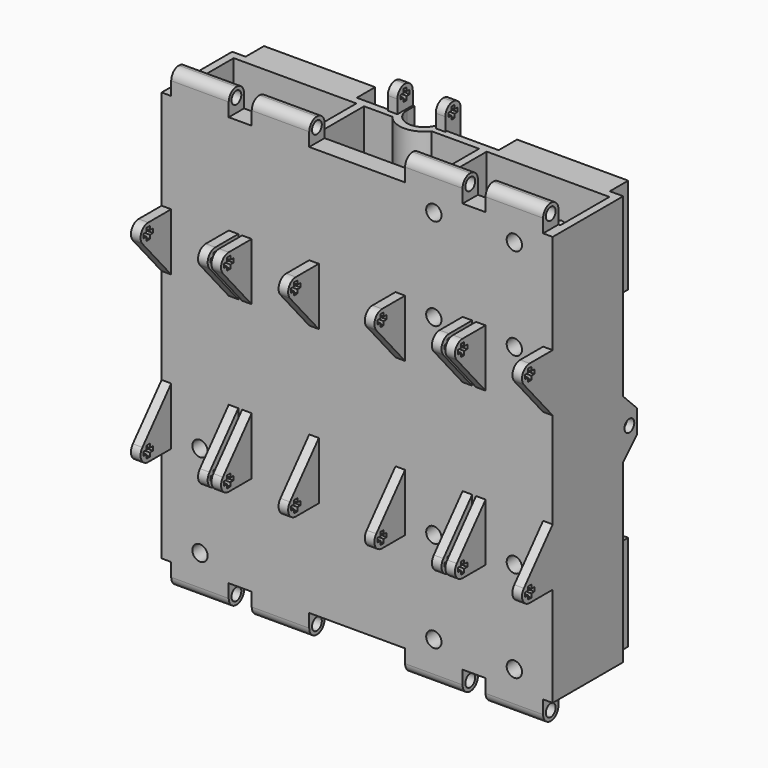
from build123d import *

# Parameters (mm, degrees)
F0_W      = 50.8
F0_H      = 25.4
F1_DEPTH  = 39.6875
F2_R      = 4.7625
F3_DEPTH  = 38.1
F5_DEPTH  = 39.6875
F6_W      = 3.96875
F6_H      = 7.9375
F7_DEPTH  = 9.525
F8_W      = 23.8125
F8_H      = 7.9375
F9_DEPTH  = 9.525
F11_DEPTH = 90.4875
F13_DEPTH = 39.6875
F14_W     = 23.8125
F14_H     = 7.9375
F14_W_2   = 3.96875
F15_DEPTH = 9.525
F16_W     = 3.96875
F16_H     = 23.8125
F17_DEPTH = 25.4
F18_R     = 3.96874
F19_R     = 3.175
F20_DEPTH = 7.9375
F21_R     = 2.54
F21_W     = 1.56845
F21_H     = 1.6891
F21_W_2   = 1.6891
F21_H_2   = 1.56845
F22_DEPTH = 161.925
F23_R     = 4.7625
F24_DEPTH = 38.1
F25_R     = 0.79375
F26_DEPTH = 3.175
F27_R     = 0.79375
F28_DEPTH = 6.35
F30_DEPTH = 39.6875
F31_R     = 1.5875
F31_R_2   = 0.79375
F32_DEPTH = 4.7625
F33_DEPTH = 3.175
F34_DEPTH = 3.175
F36_DEPTH = 161.925


# Not quite as in the source:
# - a fillet or chamfer is up to 0.001 mm smaller than in the source, because OpenCascade refuses the exact size
# - a feature names something its author has since deleted; it is built from what else it names


with BuildPart() as f1:
    # F0 (on Top) → F1 (new body)
    with BuildSketch(Plane.XY):
        Polygon((-3.175, 28.575), (-3.175, -7.9375), (158.75, -7.9375), (158.75, 28.575), (153.19375, 28.575), (153.19375, 38.1), (107.15625, 38.1), (107.15625, 28.575), (93.6625, 28.575), (93.6625, 35.71875), (69.85, 35.71875), (69.85, 28.575), (48.41875, 28.575), (48.41875, 38.1), (2.38125, 38.1), (2.38125, 28.575), align=None)
        with Locations((25.4, 12.7)):
            Rectangle(F0_W, F0_H, mode=Mode.SUBTRACT)
        Polygon((53.975, 0), (53.975, 25.4), (69.85, 25.4), (69.85, 11.6781862453), (93.6625, 11.6781862453), (93.6625, 25.4), (101.6, 25.4), (101.6, 0), align=None, mode=Mode.SUBTRACT)
        with Locations((130.175, 12.7)):
            Rectangle(F0_W, F0_H, mode=Mode.SUBTRACT)
    extrude(amount=F1_DEPTH)

    # F2 (on face) → F3 (cut)
    with BuildSketch(Plane.XY.offset(39.6875)):
        with Locations((146.84375, 31.75)):
            Circle(F2_R)
        with Locations((135.73125, 31.75)):
            Circle(F2_R)
        with Locations((113.50625, 31.75)):
            Circle(F2_R)
        with Locations((124.61875, 31.75)):
            Circle(F2_R)
        with Locations((8.73125, 31.75)):
            Circle(F2_R)
        with Locations((19.84375, 31.75)):
            Circle(F2_R)
        with Locations((30.95625, 31.75)):
            Circle(F2_R)
        with Locations((42.06875, 31.75)):
            Circle(F2_R)
    extrude(amount=-F3_DEPTH, mode=Mode.SUBTRACT)

    # F4 (on face) → F5 (cut, through all)
    with BuildSketch(Plane(origin=(0, 0, 0), x_dir=(1, 0, 0), z_dir=(0, 0, -1))):
        with BuildLine():
            Line((74.6125, -35.71875), (88.9, -35.71875))
            Line((88.9, -35.71875), (88.9, -31.75))
            ThreePointArc((88.9, -31.75), (81.75625, -24.60625), (74.6125, -31.75))
            Line((74.6125, -31.75), (74.6125, -35.71875))
        make_face()
        with BuildLine():
            Line((89.8897671705, -25.4), (93.6625, -25.4))
            Line((93.6625, -25.4), (93.6625, -11.6781862453))
            Line((93.6625, -11.6781862453), (69.85, -11.6781862453))
            Line((69.85, -11.6781862453), (69.85, -25.4))
            Line((69.85, -25.4), (73.6227328295, -25.4))
            ThreePointArc((73.6227328295, -25.4), (81.75625, -21.43125), (89.8897671705, -25.4))
        make_face()
    extrude(amount=-F5_DEPTH, mode=Mode.SUBTRACT)

    # F6 (on face) → F7 (join)
    with BuildSketch(Plane(origin=(0, 0, 0), x_dir=(1, 0, 0), z_dir=(0, 0, -1))):
        with Locations((91.678125, -31.75)):
            Rectangle(F6_W, F6_H)
        with Locations((71.834375, -31.75)):
            Rectangle(F6_W, F6_H)
    extrude(amount=F7_DEPTH)

    # F8 (on face) → F9 (join)
    with BuildSketch(Plane(origin=(0, 0, 0), x_dir=(1, 0, 0), z_dir=(0, 0, -1))):
        with Locations((142.875, 3.96875)):
            Rectangle(F8_W, F8_H)
        with Locations((12.7, 3.96875)):
            Rectangle(F8_W, F8_H)
        with Locations((109.5375, 3.96875)):
            Rectangle(F8_W, F8_H)
        with Locations((46.0375, 3.96875)):
            Rectangle(F8_W, F8_H)
    extrude(amount=F9_DEPTH)

    # F10 (on face) → F11 (join)
    with BuildSketch(Plane.XY.offset(39.6875)):
        Polygon((0, 0), (0, 35.71875), (-3.175, 35.71875), (-3.175, -7.9375), (158.75, -7.9375), (158.75, 35.71875), (155.575, 35.71875), (155.575, 0), (104.775, 0), (104.775, 35.71875), (101.6, 35.71875), (101.6, 0), (53.975, 0), (53.975, 35.71875), (50.8, 35.71875), (50.8, 0), align=None)
    extrude(amount=F11_DEPTH)

    # F12 (on face) → F13 (join)
    with BuildSketch(Plane.XY.offset(130.175)):
        Polygon((155.575, 25.4), (155.575, 28.575), (153.19375, 28.575), (153.19375, 38.1), (107.15625, 38.1), (107.15625, 28.575), (104.775, 28.575), (104.775, 25.4), align=None)
        Polygon((61.9125, 28.575), (53.975, 28.575), (53.975, 25.4), (61.9125, 25.4), (61.9125, 11.6781862453), (85.725, 11.6781862453), (85.725, 25.4), (101.6, 25.4), (101.6, 28.575), (85.725, 28.575), (85.725, 35.71875), (61.9125, 35.71875), align=None)
        Polygon((-3.175, 28.575), (-3.175, -7.9375), (158.75, -7.9375), (158.75, 28.575), (155.575, 28.575), (155.575, 25.4), (155.575, 0), (104.775, 0), (104.775, 25.4), (104.775, 28.575), (101.6, 28.575), (101.6, 25.4), (101.6, 0), (53.975, 0), (53.975, 25.4), (53.975, 28.575), (50.8, 28.575), (50.8, 25.4), (50.8, 0), (0, 0), (0, 25.4), (0, 28.575), align=None)
        Polygon((2.38125, 28.575), (0, 28.575), (0, 25.4), (50.8, 25.4), (50.8, 28.575), (48.41875, 28.575), (48.41875, 38.1), (2.38125, 38.1), align=None)
    extrude(amount=F13_DEPTH)

    # F14 (on face) → F15 (join)
    with BuildSketch(Plane.XY.offset(169.8625)):
        with Locations((12.7, -3.96875)):
            Rectangle(F14_W, F14_H)
        with Locations((109.5375, -3.96875)):
            Rectangle(F14_W, F14_H)
        with Locations((142.875, -3.96875)):
            Rectangle(F14_W, F14_H)
        with Locations((46.0375, -3.96875)):
            Rectangle(F14_W, F14_H)
        with Locations((63.896875, 31.75)):
            Rectangle(F14_W_2, F14_H)
        with Locations((83.740625, 31.75)):
            Rectangle(F14_W_2, F14_H)
    extrude(amount=F15_DEPTH)

    # F16 (on face) → F17 (join)
    with BuildSketch(Plane.XZ.offset(7.9375)):
        with Locations((156.765625, 53.18125)):
            Rectangle(F16_W, F16_H)
        with Locations((128.984375, 53.18125)):
            Rectangle(F16_W, F16_H)
        with Locations((26.590625, 53.18125)):
            Rectangle(F16_W, F16_H)
        with Locations((-1.190625, 53.18125)):
            Rectangle(F16_W, F16_H)
        with Locations((59.928125, 53.18125)):
            Rectangle(F16_W, F16_H)
        with Locations((32.146875, 53.18125)):
            Rectangle(F16_W, F16_H)
        with Locations((123.428125, 53.18125)):
            Rectangle(F16_W, F16_H)
        with Locations((95.646875, 53.18125)):
            Rectangle(F16_W, F16_H)
        with Locations((59.928125, 116.68125)):
            Rectangle(F16_W, F16_H)
        with Locations((32.146875, 116.68125)):
            Rectangle(F16_W, F16_H)
        with Locations((95.646875, 116.68125)):
            Rectangle(F16_W, F16_H)
        with Locations((123.428125, 116.68125)):
            Rectangle(F16_W, F16_H)
        with Locations((-1.190625, 116.68125)):
            Rectangle(F16_W, F16_H)
        with Locations((26.590625, 116.68125)):
            Rectangle(F16_W, F16_H)
        with Locations((156.765625, 116.68125)):
            Rectangle(F16_W, F16_H)
        with Locations((128.984375, 116.68125)):
            Rectangle(F16_W, F16_H)
    extrude(amount=F17_DEPTH)

    # F18 (radius 3.96875 in the source; OpenCascade refuses exactly that, so slightly less here)
    f18_edges = [f1.edges().sort_by_distance(p)[0] for p in [
        (91.678125, 35.71875, -9.525),
        (91.678125, 27.78125, -9.525),
        (71.834375, 35.71875, -9.525),
        (71.834375, 27.78125, -9.525),
        (142.875, 0, -9.525),
        (142.875, -7.9375, -9.525),
        (12.7, 0, -9.525),
        (12.7, -7.9375, -9.525),
        (109.5375, 0, -9.525),
        (109.5375, -7.9375, -9.525),
        (46.0375, 0, -9.525),
        (46.0375, -7.9375, -9.525),
        (12.7, 0, 179.3875),
        (12.7, -7.9375, 179.3875),
        (109.5375, 0, 179.3875),
        (142.875, 0, 179.3875),
        (109.5375, -7.9375, 179.3875),
        (142.875, -7.9375, 179.3875),
        (46.0375, 0, 179.3875),
        (46.0375, -7.9375, 179.3875),
        (63.896875, 35.71875, 179.3875),
        (63.896875, 27.78125, 179.3875),
        (83.740625, 35.71875, 179.3875),
        (83.740625, 27.78125, 179.3875),
    ]]
    fillet(f18_edges, radius=F18_R)

    # F19 (on face) → F20 (cut, through all)
    with BuildSketch(Plane.XZ.offset(7.9375)):
        with Locations((142.875, 7.14375)):
            Circle(F19_R)
        with Locations((142.875, 45.24375)):
            Circle(F19_R)
        with Locations((12.7, 45.24375)):
            Circle(F19_R)
        with Locations((12.7, 7.14375)):
            Circle(F19_R)
        with Locations((142.875, 162.71875)):
            Circle(F19_R)
        with Locations((109.5375, 162.71875)):
            Circle(F19_R)
        with Locations((109.5375, 124.61875)):
            Circle(F19_R)
        with Locations((142.875, 124.61875)):
            Circle(F19_R)
        with Locations((109.5375, 45.24375)):
            Circle(F19_R)
        with Locations((109.5375, 7.14375)):
            Circle(F19_R)
    extrude(amount=-F20_DEPTH, mode=Mode.SUBTRACT)

    # F21 (on face) → F22 (cut, through all)
    with BuildSketch(Plane.YZ.offset(158.75)):
        with Locations((-3.96875, -5.55625)):
            Circle(F21_R)
        with Locations((31.75, 84.93125)):
            Circle(F21_R)
        with Locations((30.121225, -5.55625)):
            Rectangle(F21_W, F21_H)
        with Locations((31.75, -5.55625)):
            Rectangle(F21_W_2, F21_H)
        with Locations((31.75, -7.185025)):
            Rectangle(F21_W_2, F21_H_2)
        with Locations((33.378775, -5.55625)):
            Rectangle(F21_W, F21_H)
        with Locations((31.75, -3.927475)):
            Rectangle(F21_W_2, F21_H_2)
        with BuildLine():
            Line((-22.8463210299, 47.839042618), (-7.9375, 65.0875))
            Line((-7.9375, 65.0875), (-33.3375, 65.0875))
            Line((-33.3375, 65.0875), (-33.3375, 41.275))
            Line((-33.3375, 41.275), (-19.84375, 41.275))
            ThreePointArc((-19.84375, 41.275), (-23.4528388144, 43.592854942), (-22.8463210299, 47.839042618))
        make_face()
        with Locations((-18.214975, 45.24375)):
            Rectangle(F21_W, F21_H)
        with Locations((-19.84375, 43.614975)):
            Rectangle(F21_W_2, F21_H_2)
        with Locations((-19.84375, 45.24375)):
            Rectangle(F21_W_2, F21_H)
        with Locations((-21.472525, 45.24375)):
            Rectangle(F21_W, F21_H)
        with Locations((-19.84375, 46.872525)):
            Rectangle(F21_W_2, F21_H_2)
        with Locations((-3.96875, 175.41875)):
            Circle(F21_R)
        with BuildLine():
            ThreePointArc((-22.8463210299, 122.023457382), (-23.4528388144, 126.269645058), (-19.84375, 128.5875))
            Line((-19.84375, 128.5875), (-33.3375, 128.5875))
            Line((-33.3375, 128.5875), (-33.3375, 104.775))
            Line((-33.3375, 104.775), (-7.9375, 104.775))
            Line((-7.9375, 104.775), (-22.8463210299, 122.023457382))
        make_face()
        with Locations((-21.472525, 124.61875)):
            Rectangle(F21_W, F21_H)
        with Locations((-19.84375, 124.61875)):
            Rectangle(F21_W_2, F21_H)
        with Locations((-19.84375, 122.989975)):
            Rectangle(F21_W_2, F21_H_2)
        with Locations((-18.214975, 124.61875)):
            Rectangle(F21_W, F21_H)
        with Locations((-19.84375, 126.247525)):
            Rectangle(F21_W_2, F21_H_2)
        with Locations((30.121225, 175.41875)):
            Rectangle(F21_W, F21_H)
        with Locations((31.75, 175.41875)):
            Rectangle(F21_W_2, F21_H)
        with Locations((31.75, 173.789975)):
            Rectangle(F21_W_2, F21_H_2)
        with Locations((33.378775, 175.41875)):
            Rectangle(F21_W, F21_H)
        with Locations((31.75, 177.047525)):
            Rectangle(F21_W_2, F21_H_2)
    extrude(amount=-F22_DEPTH, mode=Mode.SUBTRACT)

    # F23 (on face) → F24 (cut)
    with BuildSketch(Plane(origin=(0, 0, 130.175), x_dir=(1, 0, 0), z_dir=(0, 0, -1))):
        with Locations((146.84375, -31.75)):
            Circle(F23_R)
        with Locations((135.73125, -31.75)):
            Circle(F23_R)
        with Locations((124.61875, -31.75)):
            Circle(F23_R)
        with Locations((113.50625, -31.75)):
            Circle(F23_R)
        with Locations((8.73125, -31.75)):
            Circle(F23_R)
        with Locations((19.84375, -31.75)):
            Circle(F23_R)
        with Locations((30.95625, -31.75)):
            Circle(F23_R)
        with Locations((42.06875, -31.75)):
            Circle(F23_R)
    extrude(amount=-F24_DEPTH, mode=Mode.SUBTRACT)

    # F25 (on face) → F26 (cut)
    with BuildSketch(Plane(origin=(0, 38.1, 0), x_dir=(-1, 0, 0), z_dir=(0, 1, 0))):
        with Locations((-135.73125, 11.90625)):
            Circle(F25_R)
        with Locations((-146.84375, 11.90625)):
            Circle(F25_R)
        with Locations((-146.84375, 21.43125)):
            Circle(F25_R)
        with Locations((-135.73125, 21.43125)):
            Circle(F25_R)
        with Locations((-135.73125, 30.95625)):
            Circle(F25_R)
        with Locations((-146.84375, 30.95625)):
            Circle(F25_R)
        with Locations((-124.61875, 11.90625)):
            Circle(F25_R)
        with Locations((-124.61875, 21.43125)):
            Circle(F25_R)
        with Locations((-124.61875, 30.95625)):
            Circle(F25_R)
        with Locations((-113.50625, 11.90625)):
            Circle(F25_R)
        with Locations((-113.50625, 21.43125)):
            Circle(F25_R)
        with Locations((-113.50625, 30.95625)):
            Circle(F25_R)
        with Locations((-42.06875, 11.90625)):
            Circle(F25_R)
        with Locations((-30.95625, 11.90625)):
            Circle(F25_R)
        with Locations((-42.06875, 21.43125)):
            Circle(F25_R)
        with Locations((-30.95625, 21.43125)):
            Circle(F25_R)
        with Locations((-42.06875, 30.95625)):
            Circle(F25_R)
        with Locations((-30.95625, 30.95625)):
            Circle(F25_R)
        with Locations((-19.84375, 11.90625)):
            Circle(F25_R)
        with Locations((-8.73125, 11.90625)):
            Circle(F25_R)
        with Locations((-19.84375, 21.43125)):
            Circle(F25_R)
        with Locations((-8.73125, 21.43125)):
            Circle(F25_R)
        with Locations((-19.84375, 30.95625)):
            Circle(F25_R)
        with Locations((-8.73125, 30.95625)):
            Circle(F25_R)
        with Locations((-146.84375, 157.95625)):
            Circle(F25_R)
        with Locations((-146.84375, 148.43125)):
            Circle(F25_R)
        with Locations((-146.84375, 138.90625)):
            Circle(F25_R)
        with Locations((-135.73125, 157.95625)):
            Circle(F25_R)
        with Locations((-135.73125, 138.90625)):
            Circle(F25_R)
        with Locations((-135.73125, 148.43125)):
            Circle(F25_R)
        with Locations((-124.61875, 157.95625)):
            Circle(F25_R)
        with Locations((-124.61875, 138.90625)):
            Circle(F25_R)
        with Locations((-124.61875, 148.43125)):
            Circle(F25_R)
        with Locations((-113.50625, 157.95625)):
            Circle(F25_R)
        with Locations((-113.50625, 138.90625)):
            Circle(F25_R)
        with Locations((-113.50625, 148.43125)):
            Circle(F25_R)
    extrude(amount=-F26_DEPTH, mode=Mode.SUBTRACT)

    # F27 (on face) → F28 (cut)
    with BuildSketch(Plane.XZ.offset(-25.4)):
        with Locations((146.84375, 16.66875)):
            Circle(F27_R)
        with Locations((146.84375, 26.19375)):
            Circle(F27_R)
        with Locations((135.73125, 16.66875)):
            Circle(F27_R)
        with Locations((135.73125, 26.19375)):
            Circle(F27_R)
        with Locations((124.61875, 16.66875)):
            Circle(F27_R)
        with Locations((124.61875, 26.19375)):
            Circle(F27_R)
        with Locations((113.50625, 16.66875)):
            Circle(F27_R)
        with Locations((113.50625, 26.19375)):
            Circle(F27_R)
        with Locations((42.06875, 26.19375)):
            Circle(F27_R)
        with Locations((30.95625, 26.19375)):
            Circle(F27_R)
        with Locations((19.84375, 26.19375)):
            Circle(F27_R)
        with Locations((19.84375, 16.66875)):
            Circle(F27_R)
        with Locations((30.95625, 16.66875)):
            Circle(F27_R)
        with Locations((42.06875, 16.66875)):
            Circle(F27_R)
        with Locations((8.73125, 26.19375)):
            Circle(F27_R)
        with Locations((8.73125, 16.66875)):
            Circle(F27_R)
        with Locations((146.84375, 143.66875)):
            Circle(F27_R)
        with Locations((146.84375, 153.19375)):
            Circle(F27_R)
        with Locations((135.73125, 143.66875)):
            Circle(F27_R)
        with Locations((135.73125, 153.19375)):
            Circle(F27_R)
        with Locations((124.61875, 153.19375)):
            Circle(F27_R)
        with Locations((124.61875, 143.66875)):
            Circle(F27_R)
        with Locations((113.50625, 143.66875)):
            Circle(F27_R)
        with Locations((113.50625, 153.19375)):
            Circle(F27_R)
    extrude(amount=-F28_DEPTH, mode=Mode.SUBTRACT)

    # F29 (on face) → F30 (cut, through all)
    with BuildSketch(Plane.XY.offset(169.8625)):
        with BuildLine():
            Line((80.9625, 35.71875), (66.675, 35.71875))
            Line((66.675, 35.71875), (66.675, 31.75))
            ThreePointArc((66.675, 31.75), (73.81875, 24.60625), (80.9625, 31.75))
            Line((80.9625, 31.75), (80.9625, 35.71875))
        make_face()
        with BuildLine():
            Line((65.6852328295, 25.4), (61.9125, 25.4))
            Line((61.9125, 25.4), (61.9125, 11.6781862453))
            Line((61.9125, 11.6781862453), (85.725, 11.6781862453))
            Line((85.725, 11.6781862453), (85.725, 25.4))
            Line((85.725, 25.4), (81.9522671705, 25.4))
            ThreePointArc((81.9522671705, 25.4), (73.81875, 21.43125), (65.6852328295, 25.4))
        make_face()
    extrude(amount=-F30_DEPTH, mode=Mode.SUBTRACT)

    # F31 (on face) → F32 (join)
    with BuildSketch(Plane.XZ.offset(-25.4)):
        with Locations((146.84375, 16.66875)):
            Circle(F31_R)
        with Locations((146.84375, 16.66875)):
            Circle(F31_R_2, mode=Mode.SUBTRACT)
        with Locations((146.84375, 26.19375)):
            Circle(F31_R)
        with Locations((146.84375, 26.19375)):
            Circle(F31_R_2, mode=Mode.SUBTRACT)
        with Locations((135.73125, 26.19375)):
            Circle(F31_R)
        with Locations((135.73125, 26.19375)):
            Circle(F31_R_2, mode=Mode.SUBTRACT)
        with Locations((135.73125, 16.66875)):
            Circle(F31_R)
        with Locations((135.73125, 16.66875)):
            Circle(F31_R_2, mode=Mode.SUBTRACT)
        with Locations((124.61875, 16.66875)):
            Circle(F31_R)
        with Locations((124.61875, 16.66875)):
            Circle(F31_R_2, mode=Mode.SUBTRACT)
        with Locations((124.61875, 26.19375)):
            Circle(F31_R)
        with Locations((124.61875, 26.19375)):
            Circle(F31_R_2, mode=Mode.SUBTRACT)
        with Locations((113.50625, 16.66875)):
            Circle(F31_R)
        with Locations((113.50625, 16.66875)):
            Circle(F31_R_2, mode=Mode.SUBTRACT)
        with Locations((113.50625, 26.19375)):
            Circle(F31_R)
        with Locations((113.50625, 26.19375)):
            Circle(F31_R_2, mode=Mode.SUBTRACT)
        with Locations((113.50625, 153.19375)):
            Circle(F31_R)
        with Locations((113.50625, 153.19375)):
            Circle(F31_R_2, mode=Mode.SUBTRACT)
        with Locations((113.50625, 143.66875)):
            Circle(F31_R)
        with Locations((113.50625, 143.66875)):
            Circle(F31_R_2, mode=Mode.SUBTRACT)
        with Locations((124.61875, 153.19375)):
            Circle(F31_R)
        with Locations((124.61875, 153.19375)):
            Circle(F31_R_2, mode=Mode.SUBTRACT)
        with Locations((124.61875, 143.66875)):
            Circle(F31_R)
        with Locations((124.61875, 143.66875)):
            Circle(F31_R_2, mode=Mode.SUBTRACT)
        with Locations((135.73125, 143.66875)):
            Circle(F31_R)
        with Locations((135.73125, 143.66875)):
            Circle(F31_R_2, mode=Mode.SUBTRACT)
        with Locations((135.73125, 153.19375)):
            Circle(F31_R)
        with Locations((135.73125, 153.19375)):
            Circle(F31_R_2, mode=Mode.SUBTRACT)
        with Locations((146.84375, 153.19375)):
            Circle(F31_R)
        with Locations((146.84375, 153.19375)):
            Circle(F31_R_2, mode=Mode.SUBTRACT)
        with Locations((146.84375, 143.66875)):
            Circle(F31_R)
        with Locations((146.84375, 143.66875)):
            Circle(F31_R_2, mode=Mode.SUBTRACT)
    extrude(amount=F32_DEPTH)

    # F33 (cut): a face of the model
    f33_faces = [f1.faces().sort_by_distance(p)[0] for p in [
        (101.1027804025, 26.9875, 130.175),
    ]]
    extrude(f33_faces, amount=-F33_DEPTH, mode=Mode.SUBTRACT)

    # F34 (cut): a face of the model
    f34_faces = [f1.faces().sort_by_distance(p)[0] for p in [
        (61.9125, 28.0777804025, 39.6875),
    ]]
    extrude(f34_faces, amount=-F34_DEPTH, mode=Mode.SUBTRACT)

    # F35 (on face) → F36 (cut, through all)
    with BuildSketch(Plane(origin=(-3.175, 0, 0), x_dir=(0, -1, 0), z_dir=(-1, 0, 0))):
        Polygon((-35.71875, 130.175), (-35.71875, 89.69375), (-28.575, 96.8375), (-28.575, 130.175), align=None)
        Polygon((-35.71875, 39.6875), (-28.575, 39.6875), (-28.575, 73.025), (-35.71875, 80.16875), align=None)
    extrude(amount=-F36_DEPTH, mode=Mode.SUBTRACT)


solid = f1.part
